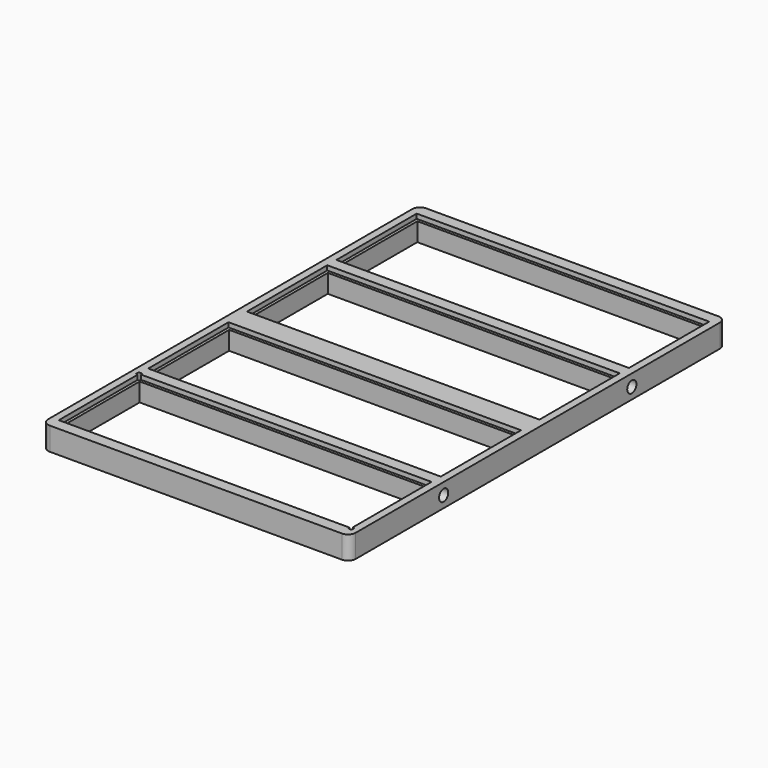
from build123d import *

# Parameters (mm, degrees)
F0_W      = 80
F0_H      = 122.4
F1_DEPTH  = 6
F2_W      = 76.1
F2_H      = 26.1
F2_W_2    = 74.6
F2_H_2    = 24.6
F3_DEPTH  = 1.2
F4_DEPTH  = 6.001
F6_D      = 3
F6_DEPTH  = 15
F6_TIP    = 0.9012909285
F8_D      = 3
F8_DEPTH  = 15
F8_TIP    = 0.9012909285
F9_R      = 2
F11_DEPTH = 6.001
F12_W     = 0.5
F12_H     = 0.5
F13_DEPTH = 4.8010001
F15_DEPTH = 6.0010001
F16_W     = 0.5
F16_H     = 0.5
F17_DEPTH = 4.8010001


# Not quite as in the source:
# - the program builds the solid bodies; features that only make, move or delete a surface that nothing else refers to are left out


with BuildPart() as f1:
    # F0 (on Top) → F1 (new body)
    with BuildSketch(Plane.XY):
        Rectangle(F0_W, F0_H)
    extrude(amount=F1_DEPTH)

    # F2 (on face) → F3 (cut)
    with BuildSketch(Plane.XY.offset(6)):
        with Locations((0, -45.15)):
            Rectangle(F2_W, F2_H)
        with Locations((0, -45.15)):
            Rectangle(F2_W_2, F2_H_2, mode=Mode.SUBTRACT)
        with Locations((0, -16.05)):
            Rectangle(F2_W, F2_H)
        with Locations((0, -16.05)):
            Rectangle(F2_W_2, F2_H_2, mode=Mode.SUBTRACT)
        with Locations((0, 16.05)):
            Rectangle(F2_W, F2_H)
        with Locations((0, 16.05)):
            Rectangle(F2_W_2, F2_H_2, mode=Mode.SUBTRACT)
        with Locations((0, 45.15)):
            Rectangle(F2_W, F2_H)
        with Locations((0, 45.15)):
            Rectangle(F2_W_2, F2_H_2, mode=Mode.SUBTRACT)
    extrude(amount=-F3_DEPTH, mode=Mode.SUBTRACT)

    # F4 (cut, through all): faces of the model
    f4_faces = [f1.faces().sort_by_distance(p)[0] for p in [
        (0, -45.15, 6),
        (0, -16.05, 6),
        (0, 16.05, 6),
        (0, 45.15, 6),
    ]]
    extrude(f4_faces, amount=-F4_DEPTH, mode=Mode.SUBTRACT)

    # F6
    with Locations(Plane.YZ.offset(40)):
        with Locations((-30.6025246664, 2.9744678242), (30.6, 2.9233971525)):
            Hole(F6_D / 2, depth=F6_DEPTH)
            with Locations((0, 0, -(F6_DEPTH + F6_TIP / 2))):  # 118° drill point
                Cone(0, F6_D / 2, F6_TIP, mode=Mode.SUBTRACT)

    # F8
    with Locations(Plane(origin=(-40, 0, 0), x_dir=(0, -1, 0), z_dir=(-1, 0, 0))):
        with Locations((30.6188296527, 2.9554700013), (-30.6144393981, 2.9124866705)):
            Hole(F8_D / 2, depth=F8_DEPTH)
            with Locations((0, 0, -(F8_DEPTH + F8_TIP / 2))):  # 118° drill point
                Cone(0, F8_D / 2, F8_TIP, mode=Mode.SUBTRACT)

    # F9
    f9_edges = [f1.edges().sort_by_distance(p)[0] for p in [
        (-40, -61.2, 3),
        (40, -61.2, 3),
        (40, 61.2, 3),
        (-40, 61.2, 3),
    ]]
    fillet(f9_edges, radius=F9_R)

    # F10 (on face) → F11 (cut, through all)
    with BuildSketch(Plane.XY.offset(6)):
        with BuildLine():
            Line((-38.3, -32.6), (-38.05, -32.6))
            Line((-38.05, -32.6), (-38.05, -32.1))
            Line((-38.05, -32.1), (-37.55, -32.1))
            Line((-37.55, -32.1), (-37.55, -31.85))
            ThreePointArc((-37.55, -31.85), (-37.6232233047, -31.6732233047), (-37.8, -31.6))
            Line((-37.8, -31.6), (-38.3, -31.6))
            ThreePointArc((-38.3, -31.6), (-38.4767766953, -31.6732233047), (-38.55, -31.85))
            Line((-38.55, -31.85), (-38.55, -32.35))
            ThreePointArc((-38.55, -32.35), (-38.4767766953, -32.5267766953), (-38.3, -32.6))
        make_face()
    extrude(amount=-F11_DEPTH, mode=Mode.SUBTRACT)

    # F12 (on face) → F13 (cut, through all)
    with BuildSketch(Plane.XY.offset(4.8)):
        with Locations((-37.8, -32.35)):
            Rectangle(F12_W, F12_H)
    extrude(amount=-F13_DEPTH, mode=Mode.SUBTRACT)

    # F14 (on face) → F15 (cut, through all)
    with BuildSketch(Plane.XY.offset(6)):
        with BuildLine():
            Line((37.8, -58.7), (38.3, -58.7))
            ThreePointArc((38.3, -58.7), (38.4767766953, -58.6267766953), (38.55, -58.45))
            Line((38.55, -58.45), (38.55, -57.95))
            ThreePointArc((38.55, -57.95), (38.4767766953, -57.7732233047), (38.3, -57.7))
            Line((38.3, -57.7), (38.05, -57.7))
            Line((38.05, -57.7), (38.05, -58.2))
            Line((38.05, -58.2), (37.55, -58.2))
            Line((37.55, -58.2), (37.55, -58.45))
            ThreePointArc((37.55, -58.45), (37.6232233047, -58.6267766953), (37.8, -58.7))
        make_face()
    extrude(amount=-F15_DEPTH, mode=Mode.SUBTRACT)

    # F16 (on face) → F17 (cut, through all)
    with BuildSketch(Plane.XY.offset(4.8)):
        with Locations((37.8, -57.95)):
            Rectangle(F16_W, F16_H)
    extrude(amount=-F17_DEPTH, mode=Mode.SUBTRACT)


solid = f1.part
